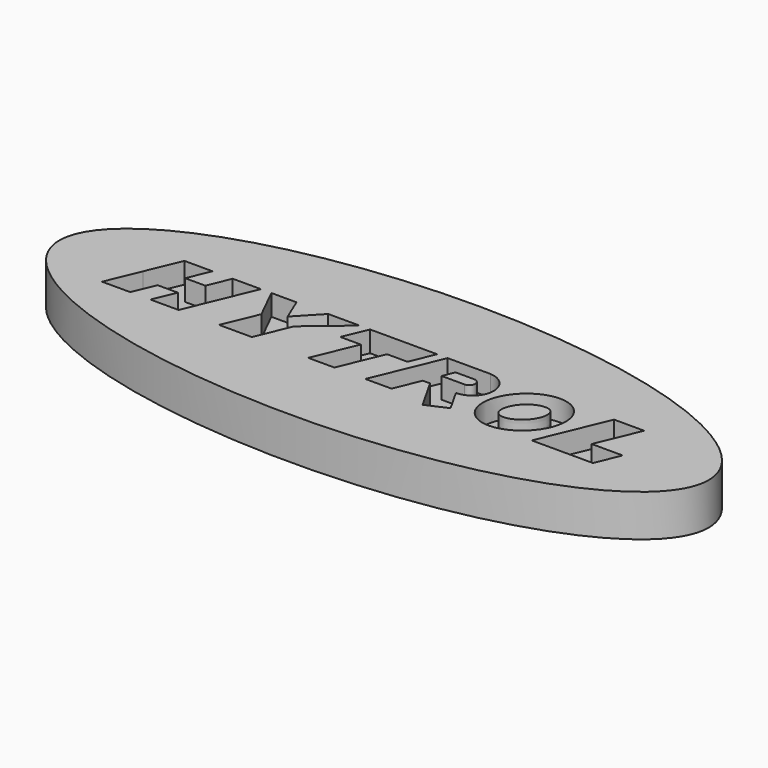
from build123d import *

# Parameters (mm, degrees)
F1_DEPTH = 12.7
F2_DEPTH = 6.35
F3_R     = 4.064
F4_DEPTH = 5.08
F5_DEPTH = 12.7


# Not quite as in the source:
# - the dataset's text gives a spline's control points without its knots; the knots are read off the source's solid
# - a feature names something its author has since deleted; it is built from what else it names


with BuildPart() as f1:
    # F0 (on Top) → F1 (new body)
    with BuildSketch(Plane.XY):
        with BuildLine():
            add(Edge.make_bspline(
                [(38.9763030052, 36.8090377465), (-59.430437785, 36.8090377465), (-59.430437785, 1.1492968171)],
                knots=[4.7123889804, 4.7123889804, 4.7123889804, 6.2831853072, 6.2831853072, 6.2831853072], degree=2, weights=[1, 0.7071067812, 1]))
            add(Edge.make_bspline(
                [(-59.430437785, 1.1492968171), (-59.430437785, -84.9409333653), (108.5603767324, -24.0659478094), (276.5511912498, 36.8090377465), (38.9763030052, 36.8090377465)],
                knots=[0, 0, 0, 2.3561944902, 2.3561944902, 4.7123889804, 4.7123889804, 4.7123889804], degree=2, weights=[1, 0.3826834324, 1, 0.3826834324, 1]))
        make_face()
        with BuildLine():
            Line((41.5160800878, -9.1104441122), (50.0543169812, 11.4090377465))
            Line((50.0543169812, 11.4090377465), (63.0317851901, 11.4090377465))
            ThreePointArc((63.0317851901, 11.4090377465), (69.090196833, 4.9107240283), (62.7350802025, -1.2977319333))
            Line((62.7350802025, -1.2977319333), (66.6440492651, -8.2119611582))
            Line((66.6440492651, -8.2119611582), (60.376466607, -10.9787322865))
            Line((60.376466607, -10.9787322865), (54.9032996575, -1.2977319333))
            Line((54.9032996575, -1.2977319333), (52.7044802725, -1.2977319333))
            Line((52.7044802725, -1.2977319333), (49.4535800878, -9.1104441122))
            Line((49.4535800878, -9.1104441122), (41.5160800878, -9.1104441122))
        make_face(mode=Mode.SUBTRACT)
        Polygon((-29.7613193382, -9.1104441122), (-38.2995562317, -9.1104441122), (-34.030437785, 1.1492968171), (-29.7613193382, 11.4090377465), (-21.2230824447, 11.4090377465), (-24.0644395016, 4.5805583649), (-17.9330891249, 4.5805583649), (-15.0917320681, 11.4090377465), (-6.5534951746, 11.4090377465), (-15.0917320681, -9.1104441122), (-23.6299689616, -9.1104441122), (-20.7886119047, -2.2819647307), (-26.9199622814, -2.2819647307), align=None, mode=Mode.SUBTRACT)
        Polygon((7.1260423387, -9.1104441122), (-2.8265984822, -9.1104441122), (1.5644947773, 1.4424322722), (-3.3784951746, 11.4090377465), (4.2415048254, 11.4090377465), (7.1743905157, 4.3774974254), (13.8377277804, 11.4090377465), (23.3627277804, 11.4090377465), (11.5171355982, 1.4424322722), align=None, mode=Mode.SUBTRACT)
        Polygon((26.5377277804, 11.4090377465), (38.9763030052, 11.4090377465), (46.8793169812, 11.4090377465), (43.7988467258, 4.0059105773), (37.5968021254, 4.0059105773), (32.1390354874, -9.1104441122), (24.2015354874, -9.1104441122), (29.6593021254, 4.0059105773), (23.457257525, 4.0059105773), align=None, mode=Mode.SUBTRACT)
        with BuildLine():
            add(Edge.make_bspline(
                [(89.9276758544, 9.4170104569), (78.4183483926, 21.1150176431), (71.5732868008, 2.8695124614), (64.7282252089, -15.3759927203), (83.0826142625, -8.8284947248), (101.4370033161, -2.2809967293), (89.9276758544, 9.4170104569)],
                knots=[0, 0, 0, 2.0943951024, 2.0943951024, 4.1887902048, 4.1887902048, 6.2831853072, 6.2831853072, 6.2831853072], degree=2, weights=[1, 0.5, 1, 0.5, 1, 0.5, 1]))
        make_face(mode=Mode.SUBTRACT)
        Polygon((91.9692541833, -9.1104441122), (100.5074910767, 11.4090377465), (109.6514910767, 11.4090377465), (104.2069794715, -1.6754618412), (113.6049794715, -1.6754618412), (110.5112541833, -9.1104441122), align=None, mode=Mode.SUBTRACT)
    extrude(amount=F1_DEPTH)

    # F0 (on Top) → F2 (join)
    with BuildSketch(Plane.XY):
        Polygon((-34.030437785, 1.1492968171), (-38.2995562317, -9.1104441122), (-29.7613193382, -9.1104441122), (-26.9199622814, -2.2819647307), (-20.7886119047, -2.2819647307), (-23.6299689616, -9.1104441122), (-15.0917320681, -9.1104441122), (-6.5534951746, 11.4090377465), (-15.0917320681, 11.4090377465), (-17.9330891249, 4.5805583649), (-24.0644395016, 4.5805583649), (-21.2230824447, 11.4090377465), (-29.7613193382, 11.4090377465), align=None)
        Polygon((1.5644947773, 1.4424322722), (-2.8265984822, -9.1104441122), (7.1260423387, -9.1104441122), (11.5171355982, 1.4424322722), (23.3627277804, 11.4090377465), (13.8377277804, 11.4090377465), (7.1743905157, 4.3774974254), (4.2415048254, 11.4090377465), (-3.3784951746, 11.4090377465), align=None)
        Polygon((46.8793169812, 11.4090377465), (38.9763030052, 11.4090377465), (26.5377277804, 11.4090377465), (23.457257525, 4.0059105773), (29.6593021254, 4.0059105773), (24.2015354874, -9.1104441122), (32.1390354874, -9.1104441122), (37.5968021254, 4.0059105773), (43.7988467258, 4.0059105773), align=None)
        with BuildLine():
            Line((63.0317851901, 11.4090377465), (50.0543169812, 11.4090377465))
            Line((50.0543169812, 11.4090377465), (41.5160800878, -9.1104441122))
            Line((41.5160800878, -9.1104441122), (49.4535800878, -9.1104441122))
            Line((49.4535800878, -9.1104441122), (52.7044802725, -1.2977319333))
            Line((52.7044802725, -1.2977319333), (54.9032996575, -1.2977319333))
            Line((54.9032996575, -1.2977319333), (62.7350802025, -1.2977319333))
            ThreePointArc((62.7350802025, -1.2977319333), (69.090196833, 4.9107240283), (63.0317851901, 11.4090377465))
        make_face()
        with BuildLine():
            Line((54.6457937759, 3.3677215688), (56.1094915291, 6.8853470303))
            Line((56.1094915291, 6.8853470303), (61.6414099932, 6.8853470303))
            ThreePointArc((61.6414099932, 6.8853470303), (63.4289023483, 5.140961916), (61.6700313985, 3.3677215688))
            Line((61.6700313985, 3.3677215688), (54.6457937759, 3.3677215688))
        make_face(mode=Mode.SUBTRACT)
        Polygon((66.6440492651, -8.2119611582), (62.7350802025, -1.2977319333), (54.9032996575, -1.2977319333), (60.376466607, -10.9787322865), align=None)
        Polygon((109.6514910767, 11.4090377465), (100.5074910767, 11.4090377465), (91.9692541833, -9.1104441122), (110.5112541833, -9.1104441122), (113.6049794715, -1.6754618412), (104.2069794715, -1.6754618412), align=None)
        with BuildLine():
            add(Edge.make_bspline(
                [(89.9276758544, 9.4170104569), (78.4183483926, 21.1150176431), (71.5732868008, 2.8695124614), (64.7282252089, -15.3759927203), (83.0826142625, -8.8284947248), (101.4370033161, -2.2809967293), (89.9276758544, 9.4170104569)],
                knots=[0, 0, 0, 2.0943951024, 2.0943951024, 4.1887902048, 4.1887902048, 6.2831853072, 6.2831853072, 6.2831853072], degree=2, weights=[1, 0.5, 1, 0.5, 1, 0.5, 1]))
        make_face()
        with BuildLine():
            add(Edge.make_bspline(
                [(85.9443699375, 5.4979521551), (85.8281310105, 5.6160966608), (85.567733934, 5.8249167649), (85.0345610289, 6.0791249218), (84.2938208293, 6.2431375515), (83.3535018874, 6.2477134028), (82.2541063192, 6.0384641997), (81.0587088146, 5.576775297), (79.8782469474, 4.8743843262), (78.7750781655, 3.9505849579), (77.8334641871, 2.8625823157), (77.1119726081, 1.6936968647), (76.630908436, 0.505964109), (76.4038115156, -0.5898838883), (76.3930978548, -1.5301529287), (76.5450449027, -2.2734619362), (76.7905504491, -2.8106976019), (77.0973883963, -3.2063344797), (77.4879840111, -3.5195646359), (78.0211569162, -3.7737727927), (78.7618971158, -3.9377854224), (79.7022160577, -3.9423612737), (80.8016116259, -3.7331120707), (81.9970091305, -3.271423168), (83.1774709977, -2.5690321972), (84.2806397796, -1.6452328289), (85.222253758, -0.5572301866), (85.943745337, 0.6116552643), (86.4248095091, 1.7993880201), (86.6519064295, 2.8952360173), (86.6626200903, 3.8355050577), (86.5106730424, 4.5788140653), (86.265167496, 5.1160497309), (86.0606088645, 5.3798076495), (85.9443699375, 5.4979521551)],
                knots=[0, 0, 0, 0, 0.03125, 0.0625, 0.09375, 0.125, 0.15625, 0.1875, 0.21875, 0.25, 0.28125, 0.3125, 0.34375, 0.375, 0.40625, 0.4375, 0.46875, 0.5, 0.53125, 0.5625, 0.59375, 0.625, 0.65625, 0.6875, 0.71875, 0.75, 0.78125, 0.8125, 0.84375, 0.875, 0.90625, 0.9375, 0.96875, 1, 1, 1, 1], degree=3))
        make_face(mode=Mode.SUBTRACT)
    extrude(amount=F2_DEPTH)

    # F3 (on face) → F4 (cut)
    with BuildSketch(Plane(origin=(0, 0, 0), x_dir=(1, 0, 0), z_dir=(0, 0, -1))):
        with Locations((3.4163030052, -1.1492968171)):
            Circle(F3_R)
        with BuildLine():
            ThreePointArc((78.6003030052, -1.1492968171), (74.5363030052, 2.9147031829), (70.4723030052, -1.1492968171))
            ThreePointArc((70.4723030052, -1.1492968171), (74.5363030052, -5.2132968171), (78.6003030052, -1.1492968171))
        make_face()
    extrude(amount=-F4_DEPTH, mode=Mode.SUBTRACT)

    # F0 (on Top) → F5 (join)
    with BuildSketch(Plane.XY):
        with BuildLine():
            Line((61.6414099932, 6.8853470303), (56.1094915291, 6.8853470303))
            Line((56.1094915291, 6.8853470303), (54.6457937759, 3.3677215688))
            Line((54.6457937759, 3.3677215688), (61.6700313985, 3.3677215688))
            ThreePointArc((61.6700313985, 3.3677215688), (63.4289023483, 5.140961916), (61.6414099932, 6.8853470303))
        make_face()
        with BuildLine():
            add(Edge.make_bspline(
                [(85.9443699375, 5.4979521551), (85.8281310105, 5.6160966608), (85.567733934, 5.8249167649), (85.0345610289, 6.0791249218), (84.2938208293, 6.2431375515), (83.3535018874, 6.2477134028), (82.2541063192, 6.0384641997), (81.0587088146, 5.576775297), (79.8782469474, 4.8743843262), (78.7750781655, 3.9505849579), (77.8334641871, 2.8625823157), (77.1119726081, 1.6936968647), (76.630908436, 0.505964109), (76.4038115156, -0.5898838883), (76.3930978548, -1.5301529287), (76.5450449027, -2.2734619362), (76.7905504491, -2.8106976019), (77.0973883963, -3.2063344797), (77.4879840111, -3.5195646359), (78.0211569162, -3.7737727927), (78.7618971158, -3.9377854224), (79.7022160577, -3.9423612737), (80.8016116259, -3.7331120707), (81.9970091305, -3.271423168), (83.1774709977, -2.5690321972), (84.2806397796, -1.6452328289), (85.222253758, -0.5572301866), (85.943745337, 0.6116552643), (86.4248095091, 1.7993880201), (86.6519064295, 2.8952360173), (86.6626200903, 3.8355050577), (86.5106730424, 4.5788140653), (86.265167496, 5.1160497309), (86.0606088645, 5.3798076495), (85.9443699375, 5.4979521551)],
                knots=[0, 0, 0, 0, 0.03125, 0.0625, 0.09375, 0.125, 0.15625, 0.1875, 0.21875, 0.25, 0.28125, 0.3125, 0.34375, 0.375, 0.40625, 0.4375, 0.46875, 0.5, 0.53125, 0.5625, 0.59375, 0.625, 0.65625, 0.6875, 0.71875, 0.75, 0.78125, 0.8125, 0.84375, 0.875, 0.90625, 0.9375, 0.96875, 1, 1, 1, 1], degree=3))
        make_face()
    extrude(amount=F5_DEPTH)


solid = f1.part
